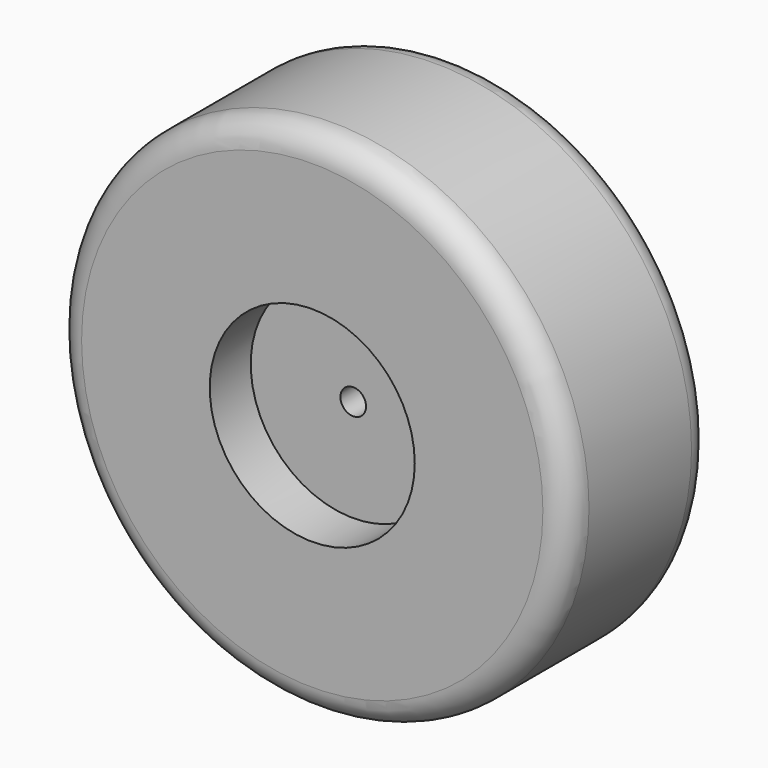
from build123d import *

# Parameters (mm, degrees)
F0_R      = 254
F1_DEPTH  = 88.9
F2_R      = 101.6
F3_DEPTH  = 63.5
F8_R      = 101.6
F9_DEPTH  = 177.8
F10_R     = 101.6
F11_DEPTH = 38.1
F12_R     = 25.4
F13_R     = 12.7
F14_DEPTH = 177.8


# Not quite as in the source:
# - a feature of the source that left no trace in its solid (it failed there, or was rolled back) is left out
# - a pattern or mirror of a feature is missing from the dataset's text; its kind, count and spacing are read off the source's solid


with BuildPart() as f1:
    # F0 (on Front) → F1 (new body, symmetric)
    with BuildSketch(Plane.XZ):
        Circle(F0_R)
    extrude(amount=F1_DEPTH, both=True)

    # F2 (on face) → F3 (cut, symmetric)
    with BuildSketch(Plane.XZ.offset(88.9)):
        Circle(F2_R)
    f3 = extrude(amount=F3_DEPTH, both=True, mode=Mode.SUBTRACT)

    # F3_copies: F3 across plane
    add(f3.mirror(Plane.ZX), mode=Mode.SUBTRACT)

    # F8 (on face) → F9 (cut, symmetric)
    with BuildSketch(Plane.XZ.offset(152.4)):
        Circle(F8_R)
    extrude(amount=F9_DEPTH, both=True, mode=Mode.SUBTRACT)

    # F10 (on Front) → F11 (join, symmetric)
    with BuildSketch(Plane.XZ):
        Circle(F10_R)
    extrude(amount=F11_DEPTH, both=True)

    # F12
    f12_edges = [f1.edges().sort_by_distance(p)[0] for p in [
        (-254, 88.9, 0),
        (-254, -88.9, 0),
    ]]
    fillet(f12_edges, radius=F12_R)

    # F13 (on face) → F14 (cut, symmetric)
    with BuildSketch(Plane(origin=(0, 38.1, 0), x_dir=(-1, 0, 0), z_dir=(0, 1, 0))):
        Circle(F13_R)
    extrude(amount=F14_DEPTH, both=True, mode=Mode.SUBTRACT)


solid = f1.part
